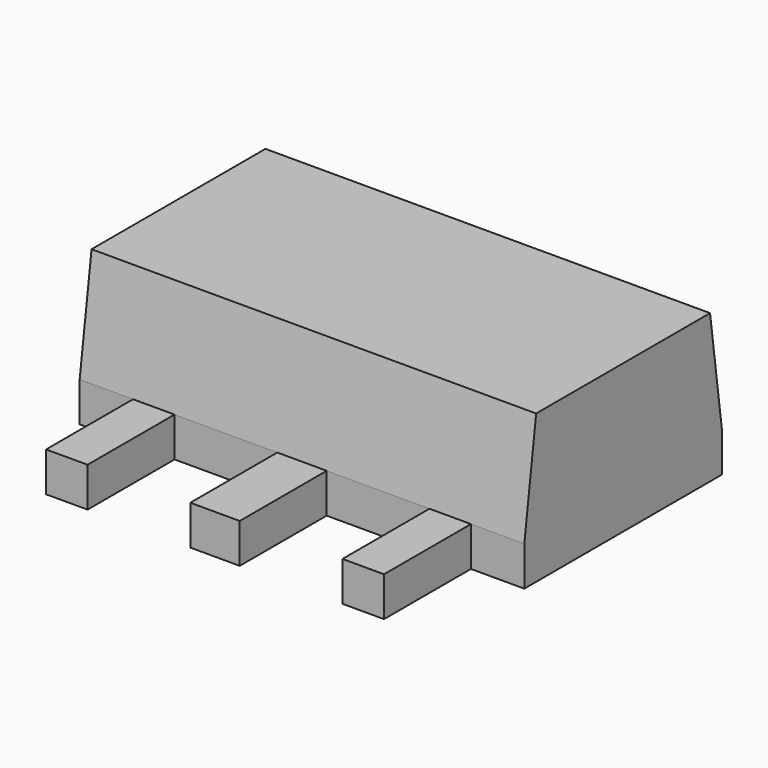
from build123d import *

# Parameters (mm, degrees)
F4_W       = 0.42
F4_H       = 1.1
F4_W_2     = 0.5
F4_H_2     = 0.7
F4_H_3     = 0.25
F4_W_3     = 1.6
F4_H_4     = 1.3
F4_H_5     = 0.5
F5_DEPTH   = 0.4
F6_DEPTH   = 0.2
F7_R       = 0.2
F8_DEPTH   = 1.5
F9_SIZE2   = 0.15
F9_SIZE    = 1.1
F9_2_SIZE2 = 0.15
F9_2_SIZE  = 1.1
F10_DEPTH  = 0.4


with BuildPart() as f5:
    # F4 (on Top) → F5 (new body)
    with BuildSketch(Plane.XY):
        with Locations((1.5, -1.8)):
            Rectangle(F4_W, F4_H)
        with Locations((0, -1.8)):
            Rectangle(F4_W_2, F4_H)
        with Locations((1.5, -0.9)):
            Rectangle(F4_W, F4_H_2)
        Polygon((0.55, -0.55), (1.29, -0.55), (1.29, -0.3), (1.71, -0.3), (1.71, -0.05), (0.8, -0.05), (0.8, -0.3), align=None)
        with Locations((1.5, -0.425)):
            Rectangle(F4_W, F4_H_3)
        with Locations((0, 0.6)):
            Rectangle(F4_W_3, F4_H_4)
        Polygon((-0.25, -1.25), (0.25, -1.25), (0.25, -0.85), (0.25, -0.55), (-0.25, -0.55), (-0.25, -0.85), align=None)
        with Locations((0, -0.425)):
            Rectangle(F4_W_2, F4_H_3)
        Polygon((0.8, -0.3), (0.8, -0.05), (-0.8, -0.05), (-0.8, -0.3), (-0.25, -0.3), (0.25, -0.3), align=None)
        with Locations((-1.5, -0.9)):
            Rectangle(F4_W, F4_H_2)
        with Locations((-1.5, -0.425)):
            Rectangle(F4_W, F4_H_3)
        Polygon((-0.8, -0.3), (-0.8, -0.05), (-1.71, -0.05), (-1.71, -0.3), (-1.29, -0.3), (-1.29, -0.55), (-0.55, -0.55), align=None)
        with Locations((-1.5, -1.8)):
            Rectangle(F4_W, F4_H)
        Polygon((-0.25, -0.3), (-0.8, -0.3), (-0.55, -0.55), (-0.25, -0.55), align=None)
        Polygon((-0.55, -0.55), (-0.25, -0.85), (-0.25, -0.55), align=None)
        Polygon((0.25, -0.55), (0.25, -0.85), (0.55, -0.55), align=None)
        Polygon((0.25, -0.55), (0.55, -0.55), (0.8, -0.3), (0.25, -0.3), align=None)
        with Locations((0, 1.5)):
            Rectangle(F4_W_3, F4_H_5)
    extrude(amount=F5_DEPTH)

    # F4 (on Top) → F6 (cut)
    with BuildSketch(Plane.XY):
        with Locations((1.5, -0.9)):
            Rectangle(F4_W, F4_H_2)
        with Locations((1.5, -0.425)):
            Rectangle(F4_W, F4_H_3)
        Polygon((0.55, -0.55), (1.29, -0.55), (1.29, -0.3), (1.71, -0.3), (1.71, -0.05), (0.8, -0.05), (0.8, -0.3), align=None)
        with Locations((-1.5, -0.9)):
            Rectangle(F4_W, F4_H_2)
        with Locations((-1.5, -0.425)):
            Rectangle(F4_W, F4_H_3)
        Polygon((-0.8, -0.3), (-0.8, -0.05), (-1.71, -0.05), (-1.71, -0.3), (-1.29, -0.3), (-1.29, -0.55), (-0.55, -0.55), align=None)
    extrude(amount=F6_DEPTH, mode=Mode.SUBTRACT)

    # F7
    f7_edges = [f5.edges().sort_by_distance(p)[0] for p in [
        (0.8, 1.75, 0.2),
        (-0.8, 1.75, 0.2),
    ]]
    fillet(f7_edges, radius=F7_R)


with BuildPart() as f8:
    # F4 (on Top) → F8 (new body)
    with BuildSketch(Plane.XY):
        Polygon((-0.8, -0.05), (-0.8, 1.25), (-2.25, 1.25), (-2.25, -1.25), (-1.71, -1.25), (-1.71, -0.55), (-1.71, -0.3), (-1.71, -0.05), align=None)
        Polygon((1.71, -1.25), (2.25, -1.25), (2.25, 1.25), (0.8, 1.25), (0.8, -0.05), (1.71, -0.05), (1.71, -0.3), (1.71, -0.55), align=None)
        with Locations((0, 0.6)):
            Rectangle(F4_W_3, F4_H_4)
        Polygon((-1.29, -1.25), (-0.25, -1.25), (-0.25, -0.85), (-0.55, -0.55), (-1.29, -0.55), align=None)
        Polygon((0.25, -1.25), (1.29, -1.25), (1.29, -0.55), (0.55, -0.55), (0.25, -0.85), align=None)
        with Locations((-1.5, -0.9)):
            Rectangle(F4_W, F4_H_2)
        with Locations((-1.5, -0.425)):
            Rectangle(F4_W, F4_H_3)
        Polygon((-0.8, -0.3), (-0.8, -0.05), (-1.71, -0.05), (-1.71, -0.3), (-1.29, -0.3), (-1.29, -0.55), (-0.55, -0.55), align=None)
        Polygon((0.8, -0.3), (0.8, -0.05), (-0.8, -0.05), (-0.8, -0.3), (-0.25, -0.3), (0.25, -0.3), align=None)
        Polygon((-0.25, -0.3), (-0.8, -0.3), (-0.55, -0.55), (-0.25, -0.55), align=None)
        Polygon((-0.25, -1.25), (0.25, -1.25), (0.25, -0.85), (0.25, -0.55), (-0.25, -0.55), (-0.25, -0.85), align=None)
        Polygon((-0.55, -0.55), (-0.25, -0.85), (-0.25, -0.55), align=None)
        with Locations((0, -0.425)):
            Rectangle(F4_W_2, F4_H_3)
        Polygon((0.25, -0.55), (0.55, -0.55), (0.8, -0.3), (0.25, -0.3), align=None)
        Polygon((0.55, -0.55), (1.29, -0.55), (1.29, -0.3), (1.71, -0.3), (1.71, -0.05), (0.8, -0.05), (0.8, -0.3), align=None)
        Polygon((0.25, -0.55), (0.25, -0.85), (0.55, -0.55), align=None)
        with Locations((1.5, -0.9)):
            Rectangle(F4_W, F4_H_2)
        with Locations((1.5, -0.425)):
            Rectangle(F4_W, F4_H_3)
    extrude(amount=F8_DEPTH)

    # F9
    f9_edges = [f8.edges().sort_by_distance(p)[0] for p in [
        (0, 1.25, 1.5),
    ]]
    f9_side = f8.faces().sort_by_distance((0, 1.25, 0.75))[0]
    chamfer(f9_edges, length=F9_SIZE, length2=F9_SIZE2, reference=f9_side)

    # F9#2
    f9_2_edges = [f8.edges().sort_by_distance(p)[0] for p in [
        (0, -1.25, 1.5),
    ]]
    f9_2_side = f8.faces().sort_by_distance((0, -1.25, 0.75))[0]
    chamfer(f9_2_edges, length=F9_2_SIZE, length2=F9_2_SIZE2, reference=f9_2_side)

    # F4 (on Top) → F10 (cut)
    with BuildSketch(Plane.XY):
        with Locations((0, 0.6)):
            Rectangle(F4_W_3, F4_H_4)
        Polygon((0.8, -0.3), (0.8, -0.05), (-0.8, -0.05), (-0.8, -0.3), (-0.25, -0.3), (0.25, -0.3), align=None)
        Polygon((-0.25, -0.3), (-0.8, -0.3), (-0.55, -0.55), (-0.25, -0.55), align=None)
        Polygon((-0.55, -0.55), (-0.25, -0.85), (-0.25, -0.55), align=None)
        Polygon((-0.25, -1.25), (0.25, -1.25), (0.25, -0.85), (0.25, -0.55), (-0.25, -0.55), (-0.25, -0.85), align=None)
        with Locations((0, -0.425)):
            Rectangle(F4_W_2, F4_H_3)
        Polygon((0.25, -0.55), (0.55, -0.55), (0.8, -0.3), (0.25, -0.3), align=None)
        Polygon((0.25, -0.55), (0.25, -0.85), (0.55, -0.55), align=None)
    extrude(amount=F10_DEPTH, mode=Mode.SUBTRACT)


solid = Compound([f5.part, f8.part])
